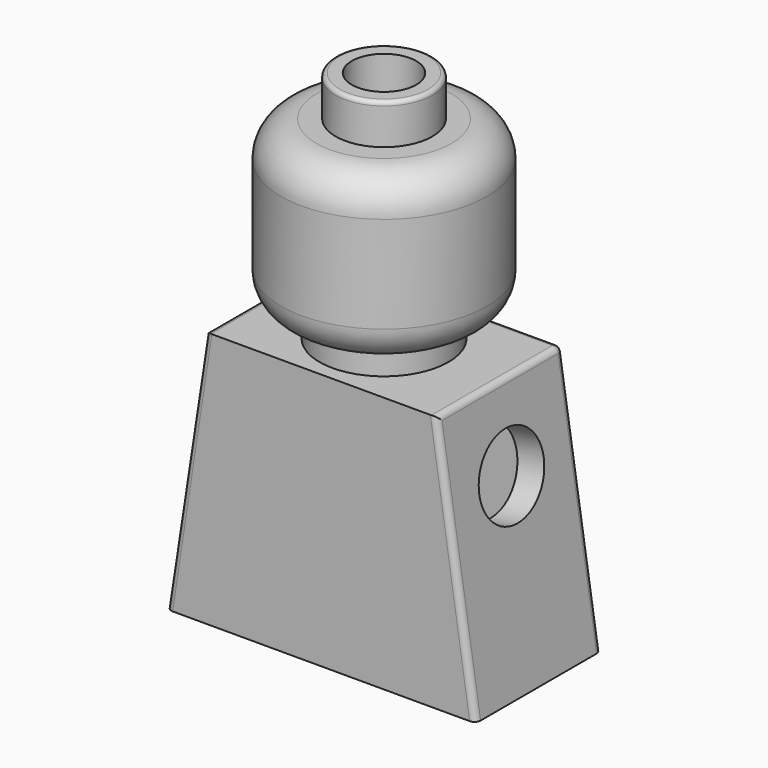
from build123d import *

# Parameters (mm, degrees)
F3_DEPTH  = 5
F4_R      = 2.4
F5_DEPTH  = 5.8
F7_DEPTH  = 3.9
F8_T      = -1.35
F11_DEPTH = 11.4
F10_R     = 2
F13_DEPTH = 1.35
F12_R     = 2
F14_DEPTH = 1.35
F15_R     = 0.3
F16_R     = 2.65
F17_DEPTH = 0.2


with BuildPart() as f1:
    # F0 (on Front) → F1 (revolve)
    with BuildSketch(Plane.XZ):
        with BuildLine():
            Line((2.5, 8.6), (2.5, 0))
            Line((2.5, 0), (3.2, 0))
            Line((3.2, 0), (3.2, 1.3))
            Line((3.2, 1.3), (3.35, 1.3))
            ThreePointArc((3.35, 1.3), (4.5874368671, 1.8125631329), (5.1, 3.05))
            Line((5.1, 3.05), (5.1, 7.85))
            ThreePointArc((5.1, 7.85), (4.5874368671, 9.0874368671), (3.35, 9.6))
            Line((3.35, 9.6), (2.4, 9.6))
            Line((2.4, 9.6), (2.4, 11.4))
            ThreePointArc((2.4, 11.4), (2.3414213562, 11.5414213562), (2.2, 11.6))
            Line((2.2, 11.6), (1.6, 11.6))
            Line((1.6, 11.6), (1.6, 9.6))
            Line((1.6, 9.6), (0, 9.6))
            Line((0, 9.6), (0, 8.6))
            Line((0, 8.6), (2.5, 8.6))
        make_face()
    revolve(axis=Axis((0, 0, 5.8), (0, 0, 1)))

    # F2 (on face) → F3 (cut)
    with BuildSketch(Plane.XY.offset(9.6)):
        with BuildLine():
            Line((-1.5491933385, 0.4), (-0.2309401077, 0.4))
            Line((-0.2309401077, 0.4), (0.4281865077, 1.5416407865))
            ThreePointArc((0.4281865077, 1.5416407865), (-0.8, 1.3856406461), (-1.5491933385, 0.4))
        make_face()
        with BuildLine():
            Line((0.4281865077, -1.5416407865), (-0.2309401077, -0.4))
            Line((-0.2309401077, -0.4), (-1.5491933385, -0.4))
            ThreePointArc((-1.5491933385, -0.4), (-0.8, -1.3856406461), (0.4281865077, -1.5416407865))
        make_face()
        with BuildLine():
            Line((1.1210068308, 1.1416407865), (0.4618802154, 0))
            Line((0.4618802154, 0), (1.1210068308, -1.1416407865))
            ThreePointArc((1.1210068308, -1.1416407865), (1.4754001032, -0.6190270878), (1.6, 0))
            ThreePointArc((1.6, 0), (1.4754001032, 0.6190270878), (1.1210068308, 1.1416407865))
        make_face()
    extrude(amount=-F3_DEPTH, mode=Mode.SUBTRACT)


with BuildPart() as f5:
    # F4 (on face) → F5 (new body)
    with BuildSketch(Plane(origin=(0, 0, 0), x_dir=(1, 0, 0), z_dir=(0, 0, -1))):
        Circle(F4_R)
    extrude(amount=-F5_DEPTH)

    # F6 (on Front) → F7 (join, symmetric)
    with BuildSketch(Plane.XZ):
        Polygon((5.725, 0), (-5.725, 0), (-7.675, -12.75), (7.675, -12.75), align=None)
    extrude(amount=F7_DEPTH, both=True)

    # F8
    f8_openings = [f5.faces().sort_by_distance(p)[0] for p in [
        (0, 0, -12.75),
    ]]
    offset(amount=F8_T, openings=f8_openings, kind=Kind.INTERSECTION)

    # F9 (on face) → F11 (join, through all)
    with BuildSketch(Plane(origin=(0, 0, -1.35), x_dir=(1, 0, 0), z_dir=(0, 0, -1))):
        Polygon((-1.625, 1.95), (-1.625, 2.55), (-2.225, 2.55), align=None)
        Polygon((2.225, 2.55), (1.625, 2.55), (1.625, 1.95), align=None)
        Polygon((1.625, -2.55), (2.225, -2.55), (1.625, -1.95), align=None)
        Polygon((-1.625, -1.95), (-2.225, -2.55), (-1.625, -2.55), align=None)
    extrude(amount=F11_DEPTH)

    # F10 (on face) → F13 (cut)
    with BuildSketch(Plane(origin=(5.5941472816, 0, 0.8555754666), x_dir=(0, 1, 0), z_dir=(0.9885057562, 0, 0.1511832333))):
        with Locations((0, -4.8655240106)):
            Circle(F10_R)
    extrude(amount=-F13_DEPTH, mode=Mode.SUBTRACT)

    # F12 (on face) → F14 (cut)
    with BuildSketch(Plane(origin=(-5.5941472816, 0, 0.8555754666), x_dir=(0, -1, 0), z_dir=(-0.9885057562, 0, 0.1511832333))):
        with Locations((0, -4.8655240106)):
            Circle(F12_R)
    extrude(amount=-F14_DEPTH, mode=Mode.SUBTRACT)

    # F15
    f15_edges = [f5.edges().sort_by_distance(p)[0] for p in [
        (-6.7, -3.9, -6.375),
        (-5.725, 0, 0),
        (-6.7, 3.9, -6.375),
        (0, 3.9, 0),
        (6.7, 3.9, -6.375),
        (5.725, 0, 0),
        (6.7, -3.9, -6.375),
    ]]
    fillet(f15_edges, radius=F15_R)


with BuildPart() as f17:
    # F16 (on face) → F17 (new body)
    with BuildSketch(Plane(origin=(-5.5941472816, 0, 0.8555754666), x_dir=(0, -1, 0), z_dir=(-0.9885057562, 0, 0.1511832333))):
        with Locations((0, -4.8655240106)):
            Circle(F16_R)
    extrude(amount=F17_DEPTH)


solid = Compound([f1.part, f5.part, f17.part])
